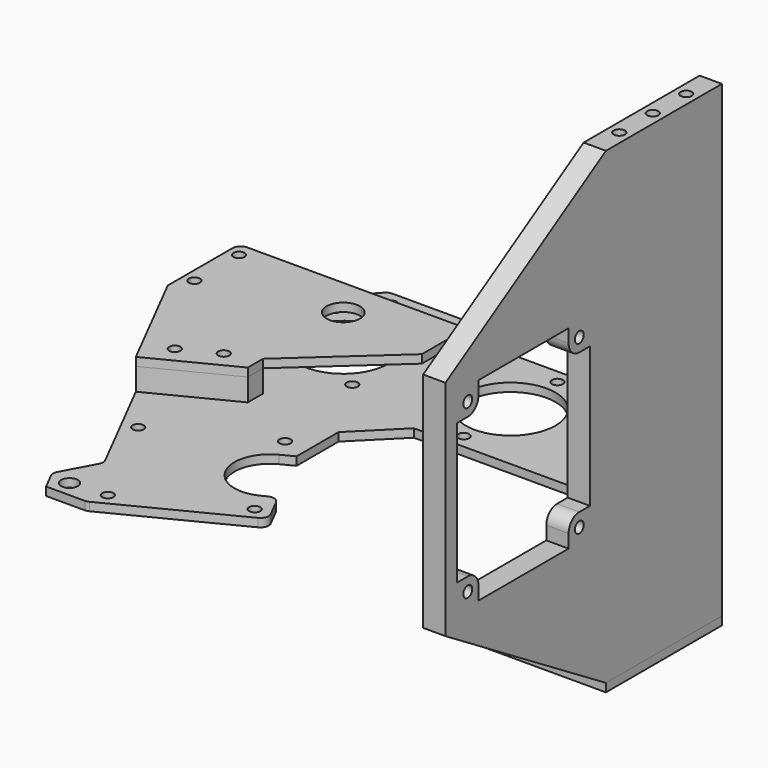
from build123d import *

# Parameters (mm, degrees)
F0_R      = 1
F0_R_2    = 1.5
F1_DEPTH  = 1.5
F2_R      = 1.5
F3_R      = 1
F3_R_2    = 8.05
F4_DEPTH  = 1.5
F5_DEPTH  = 1.5
F6_R      = 1
F7_DEPTH  = 4
F8_R      = 1
F8_R_2    = 3
F9_DEPTH  = 1.5
F10_R     = 0.8
F11_DEPTH = 4
F12_DEPTH = 5.501
F13_W     = 26
F13_H     = 1.5
F13_R     = 1
F14_DEPTH = 4
F15_R     = 1
F16_DEPTH = 1.5
F17_DEPTH = 84.001


# Not quite as in the source:
# - a feature names something its author has since deleted; it is built from what else it names


with BuildPart() as f1:
    # F0 (on Top) → F1 (new body)
    with BuildSketch(Plane.XY):
        with BuildLine():
            Line((23.5, 13), (0, 13))
            Line((0, 13), (-4, 13))
            Line((-4, 13), (-14.7961125486, 8))
            Line((-14.7961125486, 8), (-14.7961125486, -7))
            Line((-14.7961125486, -7), (2.3896440162, -40.7289463791))
            Line((2.3896440162, -40.7289463791), (4.6171603267, -39.5939701297))
            ThreePointArc((4.6171603267, -39.5939701297), (13.1578914286, -42.369021885), (10.3828396733, -50.9097529869))
            Line((10.3828396733, -50.9097529869), (8.1553233629, -52.0447292363))
            Line((8.1553233629, -52.0447292363), (11.1743601861, -57.9699226221))
            Line((11.1743601861, -57.9699226221), (34.340529815, -46.1661696289))
            Line((34.340529815, -46.1661696289), (31.3214929918, -40.240976243))
            Line((31.3214929918, -40.240976243), (29.0939766813, -41.3759524924))
            ThreePointArc((29.0939766813, -41.3759524924), (20.5532455794, -38.6009007371), (23.3282973346, -30.0601696352))
            Line((23.3282973346, -30.0601696352), (25.5558136451, -28.9251933859))
            Line((25.5558136451, -28.9251933859), (23.5, -24.8904319287))
            Line((23.5, -24.8904319287), (23.5, -13))
            Line((23.5, -13), (23.5, 13))
        make_face()
        with Locations((2.7330997527, -35.8962930544)):
            Circle(F0_R, mode=Mode.SUBTRACT)
        with Locations((12.2669002473, -54.6074300623)):
            Circle(F0_R, mode=Mode.SUBTRACT)
        with Locations((30.9780372552, -45.0736295678)):
            Circle(F0_R, mode=Mode.SUBTRACT)
        with Locations((21.4442367607, -26.3624925598)):
            Circle(F0_R, mode=Mode.SUBTRACT)
        with Locations((-12.2961125486, -4.5)):
            Circle(F0_R, mode=Mode.SUBTRACT)
        with Locations((-12.2961125486, 5.5)):
            Circle(F0_R, mode=Mode.SUBTRACT)
        Polygon((8.1553233629, -52.0447292363), (5.7264741893, -47.2778443319), (1.9778890309, -54.238311939), (3.8792396415, -57.9699226221), (11.1743601861, -57.9699226221), align=None)
        with Locations((5.7858848528, -55.1038567503)):
            Circle(F0_R_2, mode=Mode.SUBTRACT)
        Polygon((4.5558136451, 18), (0, 13), (23.5, 13), (23.5, 18), align=None)
        with Locations((7, 15.5)):
            Circle(F0_R, mode=Mode.SUBTRACT)
        with Locations((19.5, 15.5)):
            Circle(F0_R, mode=Mode.SUBTRACT)
        Polygon((23.5, 18), (23.5, 13), (25.5558136451, 13), (30.1116272902, 13), (25.5558136451, 18), align=None)
        Polygon((25.5558136451, 13), (23.5, 13), (23.5, -13), (23.5, -24.8904319287), (25.5558136451, -28.9251933859), align=None)
        Polygon((30.1116272902, 13), (25.5558136451, 13), (25.5558136451, -28.9251933859), (30.1116272902, -23.9251933859), align=None)
        with BuildLine():
            Line((4.6171603267, -39.5939701297), (2.3896440162, -40.7289463791))
            Line((2.3896440162, -40.7289463791), (5.7264741893, -47.2778443319))
            Line((5.7264741893, -47.2778443319), (8.1553233629, -52.0447292363))
            Line((8.1553233629, -52.0447292363), (10.3828396733, -50.9097529869))
            ThreePointArc((10.3828396733, -50.9097529869), (13.1578914286, -42.369021885), (4.6171603267, -39.5939701297))
        make_face()
    extrude(amount=-F1_DEPTH)

    # F2
    f2_edges = [f1.edges().sort_by_distance(p)[0] for p in [
        (5.726474, -47.277844, -0.75),
        (1.977889, -54.238312, -0.75),
        (11.17436, -57.969923, -0.75),
        (34.34053, -46.16617, -0.75),
        (30.111627, -23.925193, -0.75),
        (31.321493, -40.240976, -0.75),
        (-4, 13, -0.75),
        (-14.796113, 8, -0.75),
        (0, 13, -0.75),
        (-14.796113, -7, -0.75),
        (25.555814, 18, -0.75),
        (4.555814, 18, -0.75),
    ]]
    fillet(f2_edges, radius=F2_R)

    # F3 (on face) → F4 (join, through all)
    with BuildSketch(Plane.XY):
        Polygon((63.5, 14), (29.2004645611, 14), (30.1116272902, 13), (30.1116272902, -12), (33.0558136451, -12), (63.5, -12), align=None)
        with Locations((40, -9.5)):
            Circle(F3_R, mode=Mode.SUBTRACT)
        with Locations((61, -9.5)):
            Circle(F3_R, mode=Mode.SUBTRACT)
        with Locations((40, 1)):
            Circle(F3_R_2, mode=Mode.SUBTRACT)
        with Locations((40, 11.5)):
            Circle(F3_R, mode=Mode.SUBTRACT)
        with Locations((61, 11.5)):
            Circle(F3_R, mode=Mode.SUBTRACT)
        Polygon((33.0558136451, -12), (30.1116272902, -12), (30.1116272902, -14.9441863549), align=None)
    extrude(amount=-F4_DEPTH)

    # F3 (on face) → F5 (cut, through all)
    with BuildSketch(Plane.XY):
        with Locations((10, 1)):
            Circle(F3_R_2)
        with Locations((1.95, 9.05)):
            Circle(F3_R)
        with Locations((18.05, 9.05)):
            Circle(F3_R)
        with Locations((18.05, -7.05)):
            Circle(F3_R)
        with Locations((1.95, -7.05)):
            Circle(F3_R)
        with BuildLine():
            Line((30.1116272902, -23.3443059503), (30.1116272902, -22))
            Line((30.1116272902, -22), (30.1116272902, -14.9441863549))
            Line((30.1116272902, -14.9441863549), (25.5558136451, -19.5))
            Line((25.5558136451, -19.5), (25.5558136451, -28.9251933859))
            Line((25.5558136451, -28.9251933859), (29.7203933031, -24.3545722165))
            ThreePointArc((29.7203933031, -24.3545722165), (30.0104033658, -23.8859935819), (30.1116272902, -23.3443059503))
        make_face()
    extrude(amount=-F5_DEPTH, mode=Mode.SUBTRACT)


with BuildPart() as f7:
    # F6 (on face) → F7 (new body)
    with BuildSketch(Plane.XY):
        with BuildLine():
            Line((-8, 1), (-8, 8))
            Line((-8, 8), (-12.7961125486, 8))
            ThreePointArc((-12.7961125486, 8), (-13.8567727204, 7.5606601718), (-14.2961125486, 6.5))
            Line((-14.2961125486, 6.5), (-14.2961125486, -7.9813052528))
            Line((-14.2961125486, -7.9813052528), (-4.261316805, -27.6757007997))
            Line((-4.261316805, -27.6757007997), (10, -20.4091969443))
            Line((10, -20.4091969443), (10, -17))
            ThreePointArc((10, -17), (-2.7279220614, -11.7279220614), (-8, 1))
        make_face()
        with Locations((-12.2961125486, -4.5)):
            Circle(F6_R, mode=Mode.SUBTRACT)
        with Locations((-12.2961125486, 5.5)):
            Circle(F6_R, mode=Mode.SUBTRACT)
    extrude(amount=F7_DEPTH)

    # F10 (on face) → F11 (cut)
    with BuildSketch(Plane(origin=(-14.5780841283, -7.4279048682, 0), x_dir=(0.4539904997, -0.8910065242, 0), z_dir=(-0.8910065242, -0.4539904997, 0))):
        with Locations((16.2246326282, 2)):
            Circle(F10_R)
        with Locations((9.7246326282, 2)):
            Circle(F10_R)
        with Locations((3.2246326282, 2)):
            Circle(F10_R)
    extrude(amount=-F11_DEPTH, mode=Mode.SUBTRACT)


with BuildPart() as f9:
    # F8 (on face) → F9 (new body)
    with BuildSketch(Plane.XY.offset(4)):
        with BuildLine():
            Line((-14.2961125486, -7.9813052528), (-4.261316805, -27.6757007997))
            Line((-4.261316805, -27.6757007997), (10, -20.4091969443))
            Line((10, -20.4091969443), (10, -17))
            ThreePointArc((10, -17), (-2.7279220614, -11.7279220614), (-8, 1))
            Line((-8, 1), (-8, 8))
            Line((-8, 8), (-12.7961125486, 8))
            ThreePointArc((-12.7961125486, 8), (-13.8567727204, 7.5606601718), (-14.2961125486, 6.5))
            Line((-14.2961125486, 6.5), (-14.2961125486, -7.9813052528))
        make_face()
        with Locations((-1.5273779076, -22.3545475224)):
            Circle(F8_R, mode=Mode.SUBTRACT)
        with Locations((4.7096677618, -19.1766140242)):
            Circle(F8_R, mode=Mode.SUBTRACT)
        with Locations((-12.2961125486, -4.5)):
            Circle(F8_R, mode=Mode.SUBTRACT)
        with Locations((-12.2961125486, 5.5)):
            Circle(F8_R, mode=Mode.SUBTRACT)
        with BuildLine():
            ThreePointArc((-8, 1), (-2.7279220614, -11.7279220614), (10, -17))
            Line((10, -17), (26.5, -2))
            Line((26.5, -2), (26.5, 8))
            Line((26.5, 8), (-8, 8))
            Line((-8, 8), (-8, 1))
        make_face()
        with Locations((10, 1)):
            Circle(F8_R_2, mode=Mode.SUBTRACT)
    extrude(amount=F9_DEPTH)


with BuildPart() as f12_tool:
    # F8 (on face) → F12 (new body, through all)
    with BuildSketch(Plane.XY.offset(4)):
        with Locations((4.7096677618, -19.1766140242)):
            Circle(F8_R)
        with Locations((-1.5273779076, -22.3545475224)):
            Circle(F8_R)
    extrude(amount=-F12_DEPTH)


with BuildPart() as f1_1:
    add(f1.part)

    # F12: cut by f12_tool
    add(f12_tool.part, mode=Mode.SUBTRACT)


with BuildPart() as f7_1:
    add(f7.part)

    # F12: cut by f12_tool
    add(f12_tool.part, mode=Mode.SUBTRACT)


with BuildPart() as f14:
    # F13 (on face) → F14 (new body)
    with BuildSketch(Plane.YZ.offset(63.5)):
        with Locations((1, -0.75)):
            Rectangle(F13_W, F13_H)
        Polygon((-12, -29), (14, -29), (14, -1.5), (-12, -1.5), (-12, 0), (14, 0), (14, 55), (-12, 55), (-47.9699226221, 33), (-47.9699226221, -7), align=None)
        with Locations((-42.9699226221, -2)):
            Circle(F13_R, mode=Mode.SUBTRACT)
        with Locations((-17.9699226221, -2)):
            Circle(F13_R, mode=Mode.SUBTRACT)
        with Locations((-42.9699226221, 28)):
            Circle(F13_R, mode=Mode.SUBTRACT)
        with BuildLine():
            Line((-45.3699226221, 25.6), (-42.9699226221, 25.6))
            ThreePointArc((-42.9699226221, 25.6), (-41.2728663473, 26.3029437252), (-40.5699226221, 28))
            Line((-40.5699226221, 28), (-40.5699226221, 30.4))
            Line((-40.5699226221, 30.4), (-30.4699226221, 30.4))
            Line((-30.4699226221, 30.4), (-20.3699226221, 30.4))
            Line((-20.3699226221, 30.4), (-20.3699226221, 28))
            ThreePointArc((-20.3699226221, 28), (-19.666978897, 26.3029437252), (-17.9699226221, 25.6))
            Line((-17.9699226221, 25.6), (-15.5699226221, 25.6))
            Line((-15.5699226221, 25.6), (-15.5699226221, 13))
            Line((-15.5699226221, 13), (-15.5699226221, 0.4))
            Line((-15.5699226221, 0.4), (-17.9699226221, 0.4))
            ThreePointArc((-17.9699226221, 0.4), (-19.666978897, -0.3029437252), (-20.3699226221, -2))
            Line((-20.3699226221, -2), (-20.3699226221, -4.4))
            Line((-20.3699226221, -4.4), (-30.4699226221, -4.4))
            Line((-30.4699226221, -4.4), (-40.5699226221, -4.4))
            Line((-40.5699226221, -4.4), (-40.5699226221, -2))
            ThreePointArc((-40.5699226221, -2), (-41.2728663473, -0.3029437252), (-42.9699226221, 0.4))
            Line((-42.9699226221, 0.4), (-45.3699226221, 0.4))
            Line((-45.3699226221, 0.4), (-45.3699226221, 13))
            Line((-45.3699226221, 13), (-45.3699226221, 25.6))
        make_face(mode=Mode.SUBTRACT)
        with Locations((-17.9699226221, 28)):
            Circle(F13_R, mode=Mode.SUBTRACT)
    extrude(amount=F14_DEPTH)

    # F15 (on face) → F17 (cut, through all)
    with BuildSketch(Plane(origin=(0, 0, -29), x_dir=(1, 0, 0), z_dir=(0, 0, -1))):
        with Locations((65.5, -8.5)):
            Circle(F15_R)
        with Locations((65.5, -1)):
            Circle(F15_R)
        with Locations((65.5, 6.5)):
            Circle(F15_R)
    extrude(amount=-F17_DEPTH, mode=Mode.SUBTRACT)


with BuildPart() as f16:
    # F15 (on face) → F16 (new body)
    with BuildSketch(Plane(origin=(0, 0, -29), x_dir=(1, 0, 0), z_dir=(0, 0, -1))):
        with BuildLine():
            Line((67.5, -14), (67.5, 12))
            Line((67.5, 12), (37.5, 12))
            Line((37.5, 12), (37.5, 7.05))
            Line((37.5, 7.05), (40, 7.05))
            ThreePointArc((40, 7.05), (48.05, -1), (40, -9.05))
            Line((40, -9.05), (37.5, -9.05))
            Line((37.5, -9.05), (37.5, -14))
            Line((37.5, -14), (67.5, -14))
        make_face()
        with Locations((40, -11.5)):
            Circle(F15_R, mode=Mode.SUBTRACT)
        with Locations((61, -11.5)):
            Circle(F15_R, mode=Mode.SUBTRACT)
        with Locations((65.5, -8.5)):
            Circle(F15_R, mode=Mode.SUBTRACT)
        with Locations((40, 9.5)):
            Circle(F15_R, mode=Mode.SUBTRACT)
        with Locations((65.5, -1)):
            Circle(F15_R, mode=Mode.SUBTRACT)
        with Locations((65.5, 6.5)):
            Circle(F15_R, mode=Mode.SUBTRACT)
        with Locations((61, 9.5)):
            Circle(F15_R, mode=Mode.SUBTRACT)
    extrude(amount=F16_DEPTH)


solid = Compound([f9.part, f1_1.part, f7_1.part, f14.part, f16.part])
